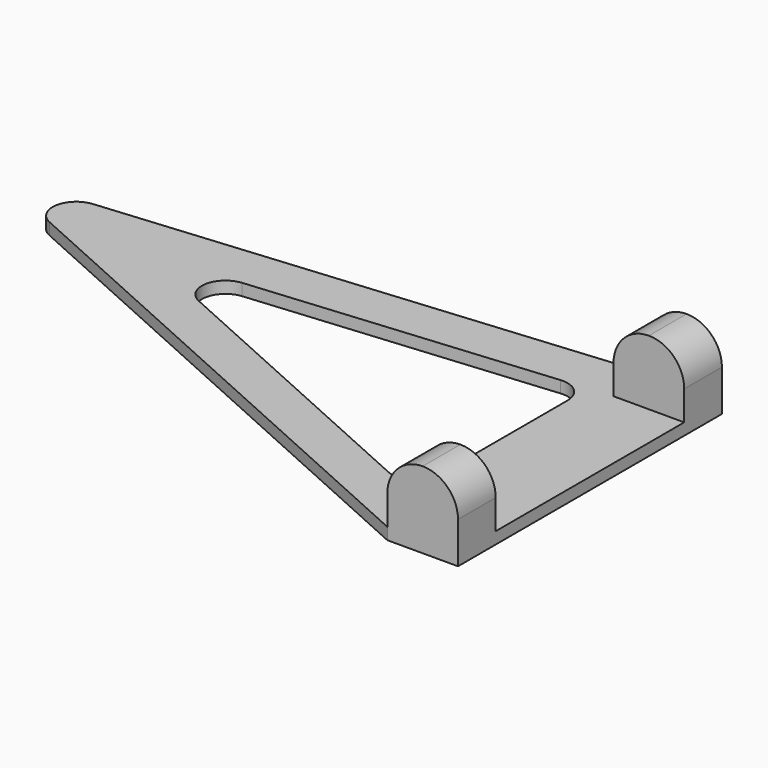
from build123d import *

# Parameters (mm, degrees)
F0_W     = 30
F0_H     = 20
F0_H_2   = 100
F1_DEPTH = 2.5
F2_DEPTH = 30
F3_R     = 14.99999


# Not quite as in the source:
# - a fillet or chamfer is up to 0.001 mm smaller than in the source, because OpenCascade refuses the exact size


with BuildPart() as f1:
    # F0 (on Top) → F1 (new body, symmetric)
    with BuildSketch(Plane.XY):
        with BuildLine():
            Line((-30, 10), (-30, 30))
            Line((-30, 30), (-250.9035135708, 9.9590995189))
            ThreePointArc((-250.9035135708, 9.9590995189), (-243.2559335601, 7.3836012794), (-240, 0))
            ThreePointArc((-240, 0), (-244.5708205421, -8.3978574895), (-254.1048020827, -9.1186950745))
            Line((-254.1048020827, -9.1186950745), (-30, -110))
            Line((-30, -110), (-30, -90))
            Line((-30, -90), (-30, 10))
        make_face()
        with BuildLine():
            ThreePointArc((-50.9035135708, 8.1035827434), (-43.2559335601, 5.5280845039), (-40, -1.8555167755))
            Line((-40, -1.8555167755), (-40, -70.0304714473))
            ThreePointArc((-40, -70.0304714473), (-44.5708205421, -78.4283289367), (-54.1048020827, -79.1491665218))
            Line((-54.1048020827, -79.1491665218), (-180.1505302804, -22.409384854))
            ThreePointArc((-180.1505302804, -22.409384854), (-185.9078460259, -11.6358085325), (-176.9492417684, -3.3315902606))
            Line((-176.9492417684, -3.3315902606), (-50.9035135708, 8.1035827434))
        make_face(mode=Mode.SUBTRACT)
        with BuildLine():
            ThreePointArc((-240, 0), (-243.2559335601, 7.3836012794), (-250.9035135708, 9.9590995189))
            ThreePointArc((-250.9035135708, 9.9590995189), (-259.8621178282, 1.654881247), (-254.1048020827, -9.1186950745))
            ThreePointArc((-254.1048020827, -9.1186950745), (-244.5708205421, -8.3978574895), (-240, 0))
        make_face()
        with Locations((-15, 20)):
            Rectangle(F0_W, F0_H)
        with Locations((-15, -40)):
            Rectangle(F0_W, F0_H_2)
        with Locations((-15, -100)):
            Rectangle(F0_W, F0_H)
    extrude(amount=F1_DEPTH, both=True)

    # F0 (on Top) → F2 (join)
    with BuildSketch(Plane.XY):
        with Locations((-15, 20)):
            Rectangle(F0_W, F0_H)
        with Locations((-15, -100)):
            Rectangle(F0_W, F0_H)
    extrude(amount=F2_DEPTH)

    # F3 (radius 15 in the source; OpenCascade refuses exactly that, so slightly less here)
    f3_edges = [f1.edges().sort_by_distance(p)[0] for p in [
        (0, 20, 30),
        (-30, 20, 30),
        (0, -100, 30),
        (-30, -100, 30),
    ]]
    fillet(f3_edges, radius=F3_R)


solid = f1.part
